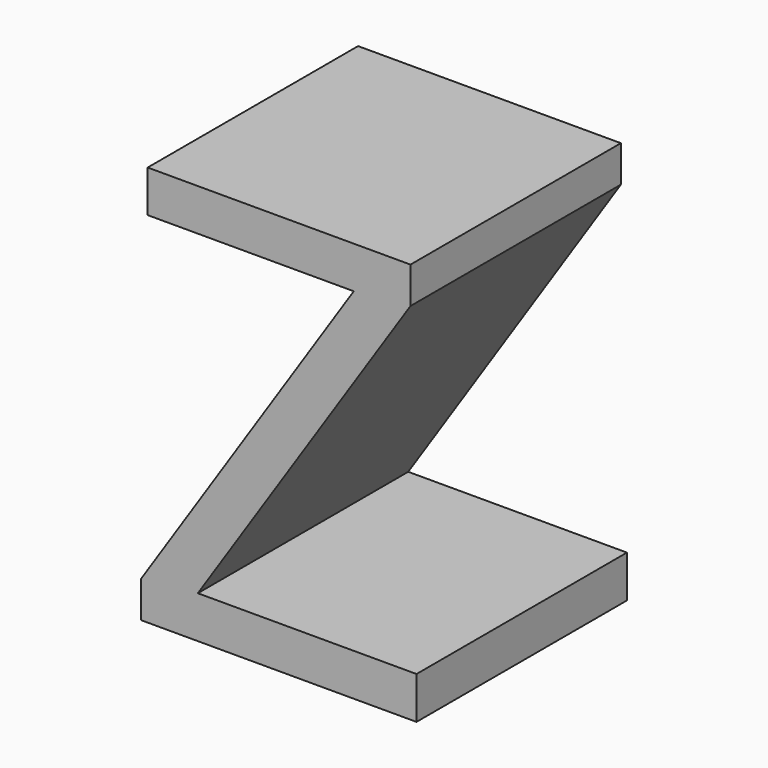
from build123d import *

# Parameters (mm, degrees)
F0_TEXT_SIZE = 54.2008814271
F1_DEPTH     = 25.4


# Not quite as in the source:
# - Text() gives the source's letters only with a copy of the font that has no kerning and outlines rounded to 1/6400 em; it was checked with that copy


with BuildPart() as f1:
    # F0 (on Front) → F1 (new body)
    with BuildSketch(Plane.XZ):
        with Locations((-17.5488116529, -16.8124997034)):
            Text('Z', F0_TEXT_SIZE, font='Open Sans', text_align=(TextAlign.LEFT, TextAlign.BOTTOM))
    extrude(amount=F1_DEPTH)


solid = f1.part
